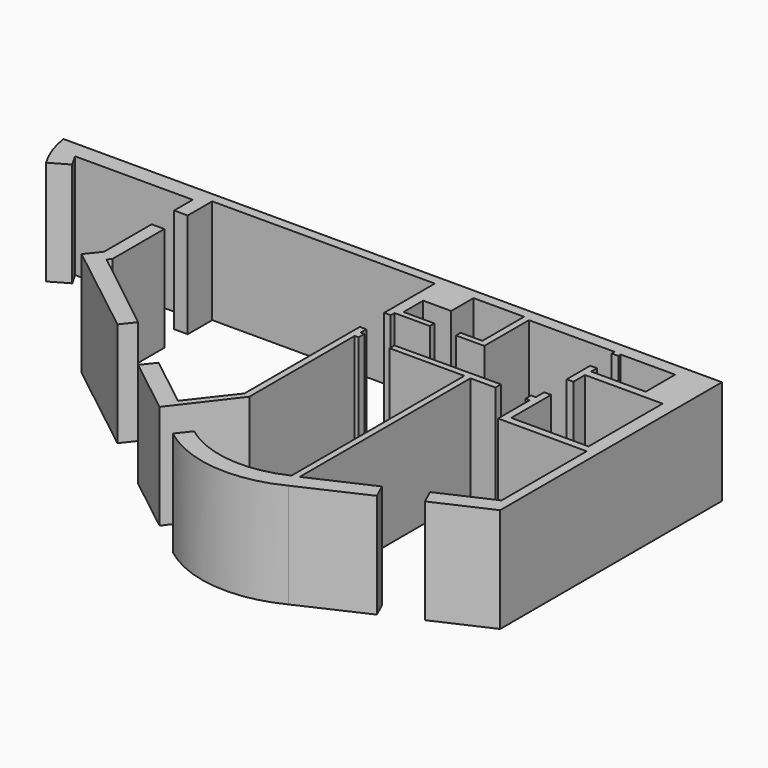
from build123d import *

# Parameters (mm, degrees)
F2_DEPTH = 2650


# Not quite as in the source:
# - a feature of the source that left no trace in its solid (it failed there, or was rolled back) is left out


with BuildPart() as f2:
    # F1 (on Top) → F2 (new body)
    with BuildSketch(Plane.XY):
        with BuildLine():
            Line((-26938.3488437603, 8660.8567436642), (-26483.4995269775, 8921.2188720703))
            Line((-26483.4995269775, 8921.2188720703), (-26661.714553833, 9232.5582504272))
            Line((-26661.714553833, 9232.5582504272), (-23679.2984008789, 9232.5582504272))
            Line((-23679.2984008789, 9232.5582504272), (-23679.2984008789, 8644.2346572876))
            Line((-23679.2984008789, 8644.2346572876), (-23335.3906952519, 8644.2346572876))
            Line((-23335.3906952519, 8644.2346572876), (-23335.3906952519, 9420.423377643))
            Line((-23335.3906952519, 9420.423377643), (-17884.4909667969, 9420.423377643))
            Line((-17884.4909667969, 9420.423377643), (-17695.3906952519, 9420.423377643))
            Line((-17695.3906952519, 9420.423377643), (-17695.3906952519, 7816.9922828674))
            Line((-17695.3906952519, 7816.9922828674), (-17529.2873382568, 7816.9922828674))
            Line((-17529.2873382568, 7816.9922828674), (-17529.2873382568, 7937.9644393921))
            Line((-17529.2873382568, 7937.9644393921), (-16637.3977661133, 7937.9644393921))
            Line((-16637.3977661133, 7937.9644393921), (-16637.3977661133, 8082.407951355))
            Line((-16637.3977661133, 8082.407951355), (-17417.3946380615, 8082.407951355))
            Line((-17417.3946380615, 8082.407951355), (-17417.3946380615, 8705.322265625))
            Line((-17417.3946380615, 8705.322265625), (-16707.8151702881, 8705.322265625))
            Line((-16707.8151702881, 8705.322265625), (-16707.8151702881, 9413.0964279175))
            Line((-16707.8151702881, 9413.0964279175), (-15427.6838302612, 9413.0964279175))
            Line((-15427.6838302612, 9413.0964279175), (-15427.6838302612, 8091.4363861084))
            Line((-15427.6838302612, 8091.4363861084), (-15980.1816940308, 8091.4363861084))
            Line((-15980.1816940308, 8091.4363861084), (-15980.1816940308, 7945.1870918274))
            Line((-15980.1816940308, 7945.1870918274), (-15261.5728378296, 7945.1870918274))
            Line((-15261.5728378296, 7945.1870918274), (-15261.5728378296, 9358.7102890015))
            Line((-15261.5728378296, 9358.7102890015), (-13094.9735641479, 9358.7102890015))
            Line((-13094.9735641479, 9358.7102890015), (-13094.9735641479, 9266.9887542725))
            Line((-13094.9735641479, 9266.9887542725), (-12923.8948822021, 9266.9887542725))
            Line((-12923.8948822021, 9266.9887542725), (-12923.8948822021, 9343.5916900635))
            Line((-12923.8948822021, 9343.5916900635), (-11542.4900054932, 9343.5916900635))
            Line((-11542.4900054932, 9343.5916900635), (-11542.4900054932, 8409.0375900269))
            Line((-11542.4900054932, 8409.0375900269), (-12923.8948822021, 8409.0375900269))
            Line((-12923.8948822021, 8409.0375900269), (-12923.8948822021, 8592.8840637207))
            Line((-12923.8948822021, 8592.8840637207), (-13094.9735641479, 8592.8840637207))
            Line((-13094.9735641479, 8592.8840637207), (-13094.9735641479, 7847.2833633423))
            Line((-13094.9735641479, 7847.2833633423), (-12926.4478683472, 7847.2833633423))
            Line((-12926.4478683472, 7847.2833633423), (-12926.4478683472, 8217.5302505493))
            Line((-12926.4478683472, 8217.5302505493), (-10960.3080749512, 8217.5302505493))
            Line((-10960.3080749512, 8217.5302505493), (-10960.3080749512, 5870.9292411804))
            Line((-10960.3080749512, 5870.9292411804), (-12918.7879562378, 5870.9292411804))
            Line((-12918.7879562378, 5870.9292411804), (-12918.7879562378, 7134.8767280579))
            Line((-12918.7879562378, 7134.8767280579), (-13094.9735641479, 7134.8767280579))
            Line((-13094.9735641479, 7134.8767280579), (-13094.9735641479, 6866.7664527893))
            Line((-13094.9735641479, 6866.7664527893), (-13212.4319076538, 6866.7664527893))
            Line((-13212.4319076538, 6866.7664527893), (-13212.4319076538, 6690.4147962649))
            Line((-13212.4319076538, 6690.4147962649), (-13106.5330505371, 6690.4147962649))
            Line((-13106.5330505371, 6690.4147962649), (-13106.5330505371, 5686.7914199829))
            Line((-13106.5330505371, 5686.7914199829), (-10858.6711883545, 5686.7914199829))
            Line((-10858.6711883545, 5686.7914199829), (-10858.6711883545, 2988.8563156128))
            Line((-10858.6711883545, 2988.8563156128), (-12186.3150742964, 2384.6693368377))
            Line((-12186.3150742964, 2384.6693368377), (-12016.0019347874, 2009.2772593156))
            Line((-12016.0019347874, 2009.2772593156), (-10618.1735992432, 2643.4636116028))
            Line((-10618.1735992432, 2643.4636116028), (-10618.1735992432, 9668.3721542358))
            Line((-10618.1735992432, 9668.3721542358), (-26876.350402832, 9668.3721542358))
            Line((-26876.350402832, 9668.3721542358), (-27302.7725219727, 9668.3721542358))
            ThreePointArc((-27302.7725219727, 9668.3721542358), (-27172.7470980576, 9145.7383452427), (-26938.3488437603, 8660.8567436642))
        make_face()
    extrude(amount=F2_DEPTH)


with BuildPart() as f2b:
    # F1 (on Top) → F2, piece 2 (new body)
    with BuildSketch(Plane.XY):
        Polygon((-23657.7911376953, 6399.5614051819), (-23941.2212371826, 6039.5283699036), (-21505.6401140405, 4130.5005509388), (-21244.5698068112, 4461.9308067403), (-23412.6605987549, 6169.7535514832), (-23335.3906952519, 6259.1233253479), (-23335.3906952519, 7903.5310745239), (-23657.7911376953, 7903.5310745239), align=None)
    extrude(amount=F2_DEPTH)


with BuildPart() as f2c:
    # F1 (on Top) → F2, piece 3 (new body)
    with BuildSketch(Plane.XY):
        Polygon((-19845.0180308134, 3359.4924935591), (-20102.637378283, 3030.8158690385), (-18647.5582122803, 1890.3132677078), (-17531.8412780762, 3343.0762290955), (-17531.8412780762, 6678.7161827087), (-17434.8106384277, 6678.7161827087), (-17434.8106384277, 6860.0096702576), (-17529.2873382568, 6860.0096702576), (-17529.2873382568, 7043.8561439514), (-17695.3906952519, 7043.8561439514), (-17695.3906952519, 3390.8414840698), (-18525.7415771484, 2320.2877044678), align=None)
    extrude(amount=F2_DEPTH)


with BuildPart() as f2d:
    # F1 (on Top) → F2, piece 4 (new body)
    with BuildSketch(Plane.XY):
        with BuildLine():
            Line((-14546.7777252197, 848.8376140594), (-12907.5493286593, 1600.5574085741))
            Line((-12907.5493286593, 1600.5574085741), (-13080.5157991396, 1977.7345856727))
            Line((-13080.5157991396, 1977.7345856727), (-14608.4012985229, 1282.4212312698))
            Line((-14608.4012985229, 1282.4212312698), (-14608.4012985229, 6690.4147962649))
            Line((-14608.4012985229, 6690.4147962649), (-13975.5125153972, 6690.4147962649))
            Line((-13975.5125153972, 6690.4147962649), (-13976.4604568481, 6865.4890060425))
            Line((-13976.4604568481, 6865.4890060425), (-16660.9916687012, 6850.953578949))
            Line((-16660.9916687012, 6850.953578949), (-16660.9916687012, 6697.7481842041))
            Line((-16660.9916687012, 6697.7481842041), (-14768.9018249512, 6697.7481842041))
            Line((-14768.9018249512, 6697.7481842041), (-14768.9018249512, 1221.9181060791))
            ThreePointArc((-14768.9018249512, 1221.9181060791), (-16153.972963618, 988.199962581), (-17460.8497619629, 1503.0972957611))
            Line((-17460.8497619629, 1503.0972957611), (-17728.5898237902, 1163.199748156))
            ThreePointArc((-17728.5898237902, 1163.199748156), (-16183.2010610926, 545.3160790761), (-14546.7777252197, 848.8376140594))
        make_face()
    extrude(amount=F2_DEPTH)


solid = Compound([f2.part, f2b.part, f2c.part, f2d.part])
